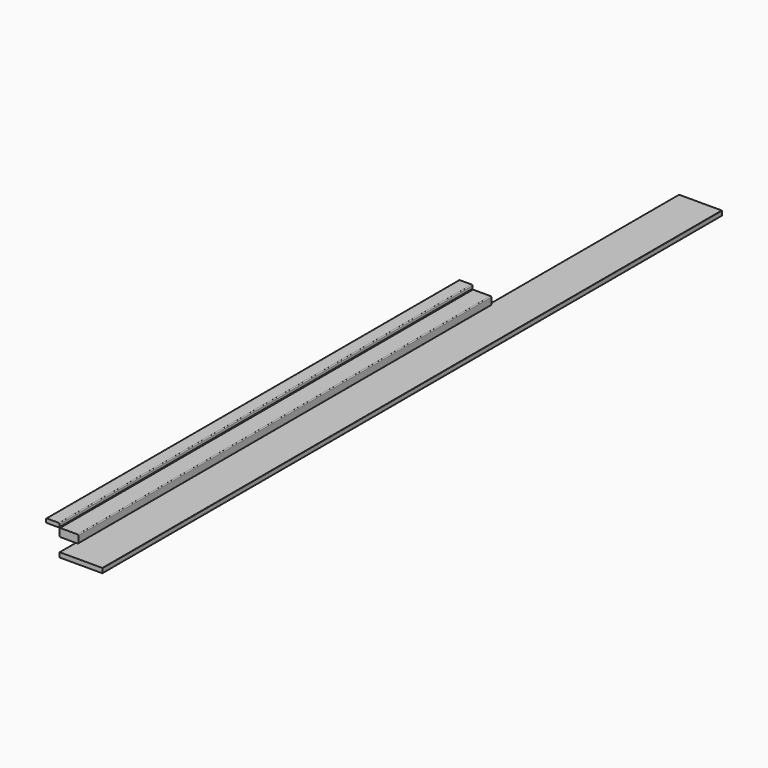
from build123d import *

# Parameters (mm, degrees)
F1_DEPTH = 2438.4
F2_DEPTH = 2438.4
F3_DEPTH = 3657.6


# Not quite as in the source:
# - a pattern or mirror of a feature is missing from the dataset's text; its kind, count and spacing are read off the source's solid


with BuildPart() as f1:
    # F0 (on Front) → F1 (new body)
    with BuildSketch(Plane.XZ):
        with BuildLine():
            Line((85.09, 0), (3.81, 0))
            ThreePointArc((3.81, 0), (1.1159231637, -1.1159231637), (0, -3.81))
            Line((0, -3.81), (0, -34.29))
            ThreePointArc((0, -34.29), (1.1159231637, -36.9840768363), (3.81, -38.1))
            Line((3.81, -38.1), (85.09, -38.1))
            ThreePointArc((85.09, -38.1), (87.7840768363, -36.9840768363), (88.9, -34.29))
            Line((88.9, -34.29), (88.9, -3.81))
            ThreePointArc((88.9, -3.81), (87.7840768363, -1.1159231637), (85.09, 0))
        make_face()
    extrude(amount=-F1_DEPTH)


with BuildPart() as f2:
    # F0 (on Front) → F2 (new body)
    with BuildSketch(Plane.XZ):
        with BuildLine():
            Line((-59.69, 0), (-3.81, 0))
            ThreePointArc((-3.81, 0), (-1.1159231637, 1.1159231637), (0, 3.81))
            Line((0, 3.81), (0, 15.24))
            ThreePointArc((0, 15.24), (-1.1159231637, 17.9340768363), (-3.81, 19.05))
            Line((-3.81, 19.05), (-59.69, 19.05))
            ThreePointArc((-59.69, 19.05), (-62.3840768363, 17.9340768363), (-63.5, 15.24))
            Line((-63.5, 15.24), (-63.5, 3.81))
            ThreePointArc((-63.5, 3.81), (-62.3840768363, 1.1159231637), (-59.69, 0))
        make_face()
    extrude(amount=-F2_DEPTH)


with BuildPart() as f3:
    # F0 (on Front) → F3 (new body)
    with BuildSketch(Plane.XZ):
        with BuildLine():
            Line((176.53, -101.6), (1.27, -101.6))
            ThreePointArc((1.27, -101.6), (0.3719743879, -101.9719743879), (0, -102.87))
            Line((0, -102.87), (0, -122.555))
            ThreePointArc((0, -122.555), (0.3719743879, -123.4530256121), (1.27, -123.825))
            Line((1.27, -123.825), (176.53, -123.825))
            ThreePointArc((176.53, -123.825), (177.4280256121, -123.4530256121), (177.8, -122.555))
            Line((177.8, -122.555), (177.8, -102.87))
            ThreePointArc((177.8, -102.87), (177.4280256121, -101.9719743879), (176.53, -101.6))
        make_face()
    extrude(amount=-F3_DEPTH)

    # F3_copies: F3 across plane


with BuildPart() as f3_1:
    add(f3.part)
    add(f3.part.mirror(Plane(origin=(101.6, 0, 0), x_dir=(0, 0, 1), z_dir=(1, 0, 0))))


solid = Compound([f1.part, f2.part, f3_1.part])
